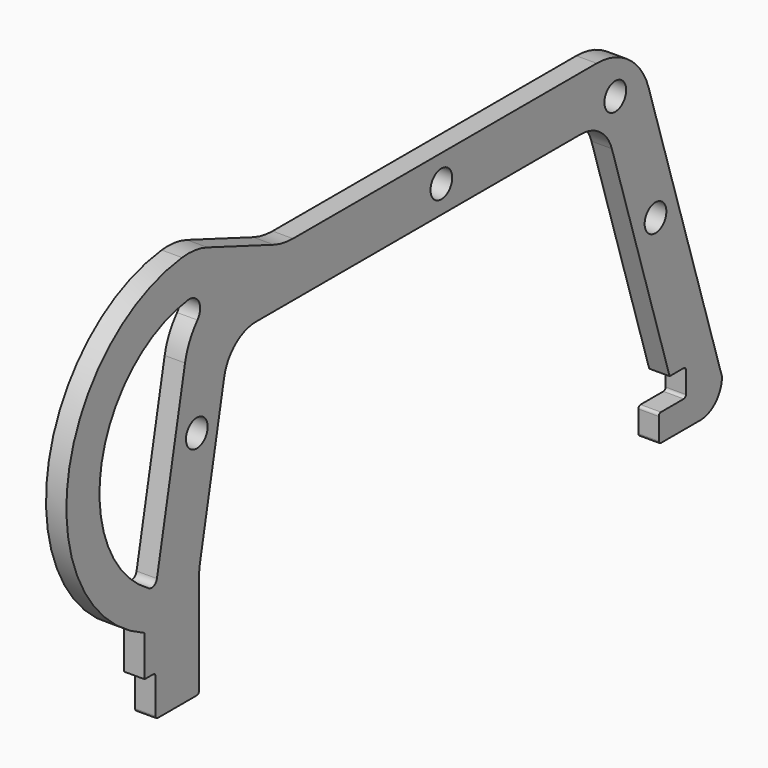
from build123d import *

# Parameters (mm, degrees)
F0_R     = 1
F1_DEPTH = 0.75


# Not quite as in the source:
# - ends of sketch curves that miss each other by under 0.0002 mm in the source are joined
# - a feature names something its author has since deleted; it is built from what else it names


with BuildPart() as f1:
    # F0 (on Right) → F1 (new body, symmetric)
    with BuildSketch(Plane.YZ):
        with BuildLine():
            Line((-22.3, -0.8), (-22.3, 6.504902432))
            ThreePointArc((-22.3, 6.504902432), (-22.2756666333, 6.9975905219), (-22.2029033785, 7.4854831077))
            Line((-22.2029033785, 7.4854831077), (-19.9823303189, 18.5883484054))
            ThreePointArc((-19.9823303189, 18.5883484054), (-18.9425550087, 20.320026424), (-17.0405882918, 21))
            Line((-17.0405882918, 21), (12.8226720923, 21))
            ThreePointArc((12.8226720923, 21), (14.5974500424, 20.4187110675), (15.6844554724, 18.9001088187))
            Line((15.6844554724, 18.9001088187), (21, 2))
            Line((21, 2), (22.3, 2))
            ThreePointArc((22.3, 2), (22.4414213562, 1.9414213562), (22.5, 1.8))
            Line((22.5, 1.8), (22.5, 0.2))
            ThreePointArc((22.5, 0.2), (22.4414213562, 0.0585786438), (22.3, 0))
            Line((22.3, 0), (20.2, 0))
            ThreePointArc((20.2, 0), (20.0585786438, -0.0585786438), (20, -0.2))
            Line((20, -0.2), (20, -1.8))
            ThreePointArc((20, -1.8), (20.0585786438, -1.9414213562), (20.2, -2))
            Line((20.2, -2), (23.8107259146, -2))
            ThreePointArc((23.8107259146, -2), (25.2243140233, -1.4148387396), (25.8107251326, -0.001768659))
            ThreePointArc((25.8107251326, -0.001768659), (25.8107257191, -0.0008843296), (25.8107259146, 0))
            ThreePointArc((25.8107259146, 0), (25.8076938609, 0.0370492941), (25.799207863, 0.0732404086))
            Line((25.799207863, 0.0732404086), (19.059851332, 21.5001813645))
            ThreePointArc((19.059851332, 21.5001813645), (17.2481756153, 24.0311851125), (14.2902123652, 25))
            Line((14.2902123652, 25), (-13.6493669984, 25))
            ThreePointArc((-13.6493669984, 25), (-14.5478772467, 25.0813945743), (-15.4171339514, 25.3229282665))
            Line((-15.4171339514, 25.3229282665), (-21.5261195006, 27.6319077703))
            ThreePointArc((-21.5261195006, 27.6319077703), (-22.6761929546, 27.9165348126), (-23.8609482061, 27.9225760631))
            ThreePointArc((-23.8609482061, 27.9225760631), (-34.3671649706, 17.7805604622), (-27.3, 5.0018183321))
            Line((-27.3, 5.0018183321), (-27.3, 2))
            Line((-27.3, 2), (-26.5, 2))
            ThreePointArc((-26.5, 2), (-26.3585786438, 1.9414213562), (-26.3, 1.8))
            Line((-26.3, 1.8), (-26.3, -0.8))
            ThreePointArc((-26.3, -0.8), (-26.2414213562, -0.9414213562), (-26.1, -1))
            Line((-26.1, -1), (-22.5, -1))
            ThreePointArc((-22.5, -1), (-22.3585786438, -0.9414213562), (-22.3, -0.8))
        make_face()
        with Locations((19.6997005895, 12.8)):
            Circle(F0_R, mode=Mode.SUBTRACT)
        with BuildLine():
            Line((-23.5830994757, 20.9805806757), (-26.1667940449, 8.0621078301))
            ThreePointArc((-26.1667940449, 8.0621078301), (-26.4540531191, 7.7032432499), (-26.9129154865, 7.7305725477))
            ThreePointArc((-26.9129154865, 7.7305725477), (-31.2579507019, 17.6226927508), (-23.3162298506, 24.9481581324))
            ThreePointArc((-23.3162298506, 24.9481581324), (-22.308062771, 24.4249028415), (-22.4394560446, 23.2966596198))
            ThreePointArc((-22.4394560446, 23.2966596198), (-23.1634230366, 22.2137470973), (-23.5830994757, 20.9805806757))
        make_face(mode=Mode.SUBTRACT)
        with Locations((-22.5, 16)):
            Circle(F0_R, mode=Mode.SUBTRACT)
        with Locations((0, 23)):
            Circle(F0_R, mode=Mode.SUBTRACT)
        with Locations((16, 22.1668636565)):
            Circle(F0_R, mode=Mode.SUBTRACT)
    extrude(amount=F1_DEPTH, both=True)


solid = f1.part
